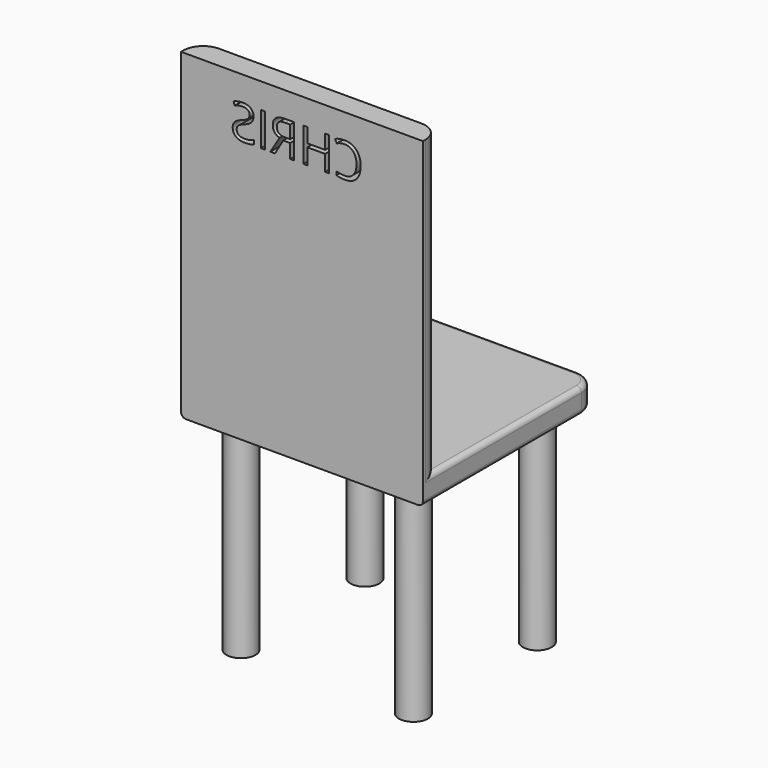
from build123d import *

# Parameters (mm, degrees)
F1_DEPTH     = 25
F3_DEPTH     = 300
F4_R         = 14.6144716814
F5_DEPTH     = 208
F6_R         = 5
F7_TEXT_SIZE = 47.7535857095
F8_DEPTH     = 22.8913672099


# Not quite as in the source:
# - Text() gives the source's letters only with a copy of the font that has no kerning and outlines rounded to 1/6400 em; it was checked with that copy


with BuildPart() as f1:
    # F0 (on Top) → F1 (new body)
    with BuildSketch(Plane.XY):
        with BuildLine():
            Line((-122.1492225489, -110), (122.1492225489, -110))
            Line((122.1492225489, -110), (122.1492225489, 90))
            ThreePointArc((122.1492225489, 90), (116.2913581726, 104.1421356237), (102.1492225489, 110))
            Line((102.1492225489, 110), (-102.1492225489, 110))
            ThreePointArc((-102.1492225489, 110), (-116.2913581726, 104.1421356237), (-122.1492225489, 90))
            Line((-122.1492225489, 90), (-122.1492225489, -110))
        make_face()
    extrude(amount=F1_DEPTH)

    # F2 (on face) → F3 (join)
    with BuildSketch(Plane.XY.offset(25)):
        with BuildLine():
            Line((-122.1492225489, -107.1096327901), (-122.1492225489, -110))
            Line((-122.1492225489, -110), (122.1492225489, -110))
            Line((122.1492225489, -110), (122.1492225489, -107.1096327901))
            ThreePointArc((122.1492225489, -107.1096327901), (116.2913581726, -92.9674971664), (102.1492225489, -87.1096327901))
            Line((102.1492225489, -87.1096327901), (-102.1492225489, -87.1096327901))
            ThreePointArc((-102.1492225489, -87.1096327901), (-116.2913581726, -92.9674971664), (-122.1492225489, -107.1096327901))
        make_face()
    extrude(amount=F3_DEPTH)

    # F4 (on face) → F5 (join)
    with BuildSketch(Plane(origin=(0, 0, 0), x_dir=(1, 0, 0), z_dir=(0, 0, -1))):
        with Locations((-87.0373249054, -78.1772062182)):
            Circle(F4_R)
        with Locations((87.0373249054, -78.1772062182)):
            Circle(F4_R)
        with Locations((87.0373249054, 78.1772062182)):
            Circle(F4_R)
        with Locations((-87.0373249054, 78.1772062182)):
            Circle(F4_R)
    extrude(amount=F5_DEPTH)

    # F6
    f6_edges = [f1.edges().sort_by_distance(p)[0] for p in [
        (0, 110, 25),
        (0, 110, 0),
    ]]
    fillet(f6_edges, radius=F6_R)

    # F7 (on face) → F8 (cut, through all)
    with BuildSketch(Plane(origin=(0, -87.1096327901, 0), x_dir=(-1, 0, 0), z_dir=(0, 1, 0))):
        with Locations((-62.1357485652, 265.5180692673)):
            Text('CHRIS', F7_TEXT_SIZE, font='Open Sans', text_align=(TextAlign.LEFT, TextAlign.BOTTOM))
    extrude(amount=-F8_DEPTH, mode=Mode.SUBTRACT)


solid = f1.part
